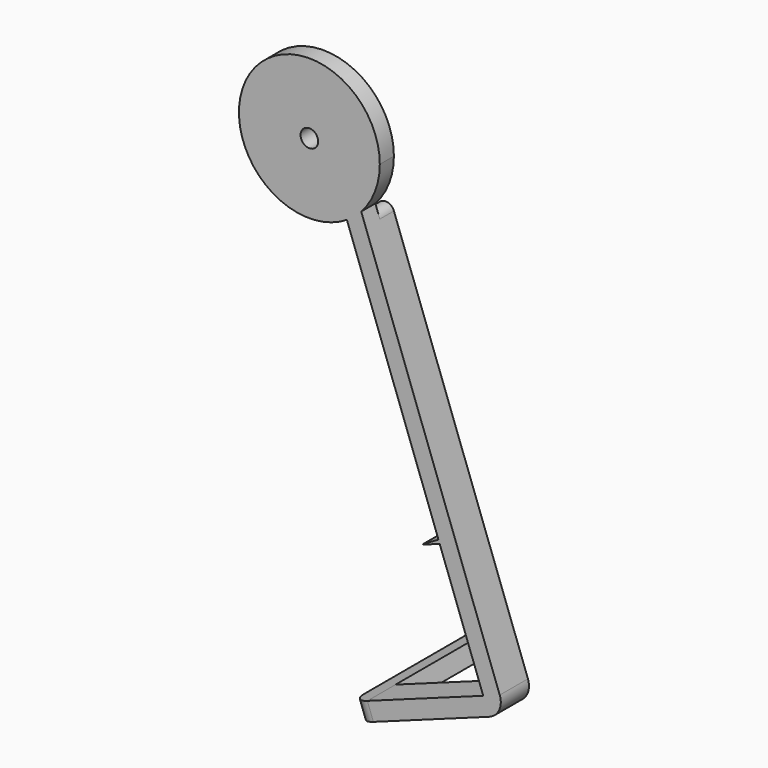
from build123d import *

# Parameters (mm, degrees)
F0_R     = 2.5
F1_DEPTH = 5
F2_DEPTH = 5
F3_R     = 4.99999
F4_R     = 2.49999
F5_SIZE2 = 0.881625
F5_SIZE  = 4.99999
F6_DEPTH = 40


# Not quite as in the source:
# - a fillet or chamfer is up to 0.001 mm smaller than in the source, because OpenCascade refuses the exact size
# - a feature names something its author has since deleted; it is built from what else it names


with BuildPart() as f1:
    # F0 (on Front) → F1 (new body)
    with BuildSketch(Plane.XZ):
        with BuildLine():
            ThreePointArc((14.7291057085, 20.287369527), (18.6357467541, 26.5570015397), (20, 33.8170940264))
            ThreePointArc((20, 33.8170940264), (-17.5060505822, 43.4886085414), (10.6461806987, 16.8860917959))
            ThreePointArc((10.6461806987, 16.8860917959), (12.8011117725, 18.4505219497), (14.7291057085, 20.287369527))
        make_face()
        with Locations((0, 33.8170940264)):
            Circle(F0_R, mode=Mode.SUBTRACT)
        Polygon((18.1838180761, -106.1565507003), (51.0730598036, -94.1858456839), (49.362959087, -89.48738258), (16.4737173595, -101.4580875964), align=None)
        Polygon((13.4853549722, -107.8666514169), (18.1838180761, -106.1565507003), (16.4737173595, -101.4580875964), (11.7752542555, -103.168188313), align=None)
        Polygon((37.0066776717, -55.538778403), (36.6646575283, -54.5990857822), (31.9661944244, -56.3091864988), (32.3082145677, -57.2488791196), align=None)
        with BuildLine():
            ThreePointArc((14.7291057085, 20.287369527), (12.8011117725, 18.4505219497), (10.6461806987, 16.8860917959))
            Line((10.6461806987, 16.8860917959), (36.6646575283, -54.5990857822))
            Line((36.6646575283, -54.5990857822), (37.0066776717, -55.538778403))
            Line((37.0066776717, -55.538778403), (49.362959087, -89.48738258))
            Line((49.362959087, -89.48738258), (51.0730598036, -94.1858456839))
            Line((51.0730598036, -94.1858456839), (55.7715229075, -92.4757449673))
            Line((55.7715229075, -92.4757449673), (14.7291057085, 20.287369527))
        make_face()
    extrude(amount=F1_DEPTH)

    # F0 (on Front) → F2 (join)
    with BuildSketch(Plane.XZ):
        Polygon((37.0066776717, -55.538778403), (36.6646575283, -54.5990857822), (31.9661944244, -56.3091864988), (32.3082145677, -57.2488791196), align=None)
        with BuildLine():
            ThreePointArc((14.7291057085, 20.287369527), (12.8011117725, 18.4505219497), (10.6461806987, 16.8860917959))
            Line((10.6461806987, 16.8860917959), (36.6646575283, -54.5990857822))
            Line((36.6646575283, -54.5990857822), (37.0066776717, -55.538778403))
            Line((37.0066776717, -55.538778403), (49.362959087, -89.48738258))
            Line((49.362959087, -89.48738258), (51.0730598036, -94.1858456839))
            Line((51.0730598036, -94.1858456839), (55.7715229075, -92.4757449673))
            Line((55.7715229075, -92.4757449673), (14.7291057085, 20.287369527))
        make_face()
        Polygon((18.1838180761, -106.1565507003), (51.0730598036, -94.1858456839), (49.362959087, -89.48738258), (16.4737173595, -101.4580875964), align=None)
    extrude(amount=-F2_DEPTH)

    # F3 (radius 5 in the source; OpenCascade refuses exactly that, so slightly less here)
    f3_edges = [f1.edges().sort_by_distance(p)[0] for p in [
        (55.771523, 0, -92.475745),
        (12.630305, -5, -105.51742),
    ]]
    fillet(f3_edges, radius=F3_R)

    # F4 (radius 2.5 in the source; OpenCascade refuses exactly that, so slightly less here)
    f4_edges = [f1.edges().sort_by_distance(p)[0] for p in [
        (14.729106, 2.5, 20.28737),
        (10.646181, 2.5, 16.886092),
    ]]
    fillet(f4_edges, radius=F4_R)

    # F5 (size 5 and 0.8816349035 in the source; OpenCascade refuses exactly that, so slightly less here)
    f5_edges = [f1.edges().sort_by_distance(p)[0] for p in [
        (31.966194, 0, -56.309186),
    ]]
    chamfer(f5_edges, length=F5_SIZE, length2=F5_SIZE2)

    # F0 (on Front) → F6 (join)
    with BuildSketch(Plane.XZ):
        Polygon((13.4853549722, -107.8666514169), (18.1838180761, -106.1565507003), (16.4737173595, -101.4580875964), (11.7752542555, -103.168188313), align=None)
    extrude(amount=-F6_DEPTH)


solid = f1.part
